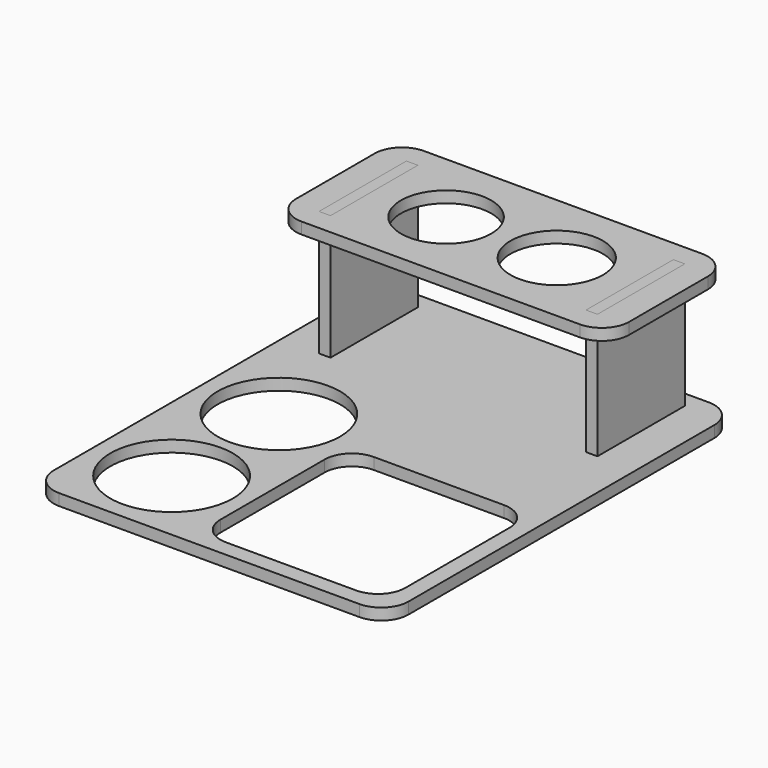
from build123d import *

# Parameters (mm, degrees)
F1_W     = 165.1
F1_H     = 203.2
F1_R     = 28.5
F1_W_2   = 86.0044
F1_H_2   = 86
F1_W_3   = 5.334
F1_H_3   = 50.8
F2_DEPTH = 5.334
F3_W     = 5.334
F3_H     = 50.8
F4_DEPTH = 63.5
F5_W     = 154.94
F5_H     = 71.12
F5_W_2   = 5.334
F5_H_2   = 50.8
F5_R     = 21.5
F5_R_2   = 21
F6_DEPTH = 5.334
F7_R     = 12.7
F7_2_R   = 12.7


# Not quite as in the source:
# - a variable given as a bare number and used for a length is read in inches; the dataset says mm whatever the document's units were


with BuildPart() as f2:
    # F1 (on Top) → F2 (new body)
    with BuildSketch(Plane.XY):
        Rectangle(F1_W, F1_H)
        with Locations((-46.43, -65.48)):
            Circle(F1_R, mode=Mode.SUBTRACT)
        with Locations((-46.4312, -3.1)):
            Circle(F1_R, mode=Mode.SUBTRACT)
        with Locations((31.9278, -50.98)):
            Rectangle(F1_W_2, F1_H_2, mode=Mode.SUBTRACT)
        with Locations((-62.103, 68.58)):
            Rectangle(F1_W_3, F1_H_3, mode=Mode.SUBTRACT)
        with Locations((62.103, 68.58)):
            Rectangle(F1_W_3, F1_H_3, mode=Mode.SUBTRACT)
    extrude(amount=F2_DEPTH)

    # F7
    f7_edges = [f2.edges().sort_by_distance(p)[0] for p in [
        (-82.55, -101.6, 2.667),
        (82.55, -101.6, 2.667),
        (-82.55, 101.6, 2.667),
        (82.55, 101.6, 2.667),
        (-11.0744, -7.98, 2.667),
        (74.93, -7.98, 2.667),
        (74.93, -93.98, 2.667),
        (-11.0744, -93.98, 2.667),
    ]]
    fillet(f7_edges, radius=F7_R)


with BuildPart() as f4:
    # F3 (on face) → F4 (new body)
    with BuildSketch(Plane(origin=(0, 0, 0), x_dir=(1, 0, 0), z_dir=(0, 0, -1))):
        with Locations((-62.103, -68.58)):
            Rectangle(F3_W, F3_H)
    extrude(amount=-F4_DEPTH)


with BuildPart() as f4b:
    # F3 (on face) → F4, piece 2 (new body)
    with BuildSketch(Plane(origin=(0, 0, 0), x_dir=(1, 0, 0), z_dir=(0, 0, -1))):
        with Locations((62.103, -68.58)):
            Rectangle(F3_W, F3_H)
    extrude(amount=-F4_DEPTH)


with BuildPart() as f6:
    # F5 (on face) → F6 (new body)
    with BuildSketch(Plane.XY.offset(63.5)):
        with Locations((0, 68.58)):
            Rectangle(F5_W, F5_H)
        with Locations((-62.103, 68.58)):
            Rectangle(F5_W_2, F5_H_2, mode=Mode.SUBTRACT)
        with Locations((25.49, 68.5789)):
            Circle(F5_R, mode=Mode.SUBTRACT)
        with Locations((62.103, 68.58)):
            Rectangle(F5_W_2, F5_H_2, mode=Mode.SUBTRACT)
        with Locations((-25.99, 68.5858)):
            Circle(F5_R_2, mode=Mode.SUBTRACT)
    extrude(amount=-F6_DEPTH)

    # F7#2
    f7_2_edges = [f6.edges().sort_by_distance(p)[0] for p in [
        (-77.47, 33.02, 60.833),
        (-77.47, 104.14, 60.833),
        (77.47, 33.02, 60.833),
        (77.47, 104.14, 60.833),
    ]]
    fillet(f7_2_edges, radius=F7_2_R)


solid = Compound([f2.part, f4.part, f4b.part, f6.part])
